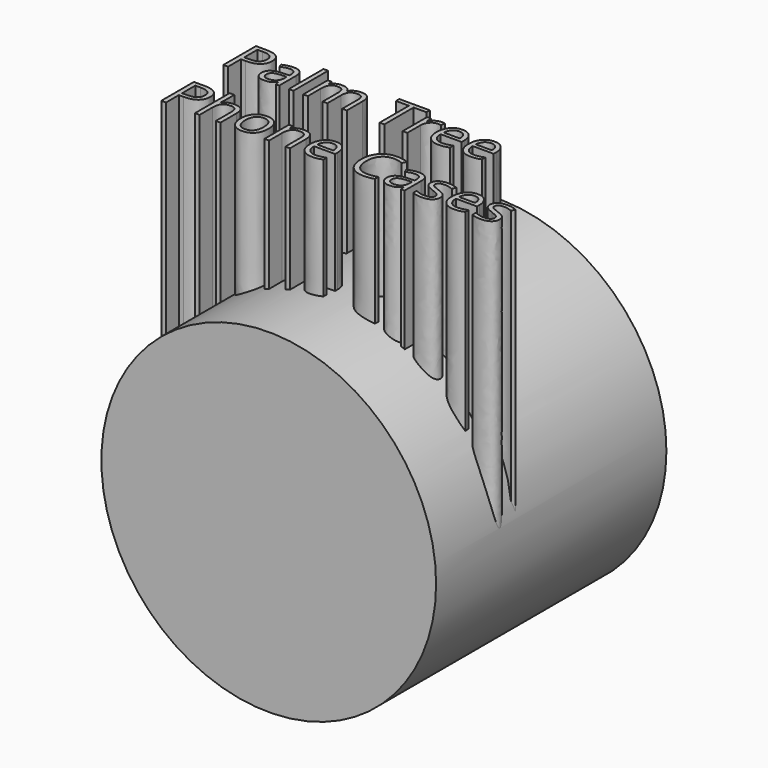
from build123d import *

# Parameters (mm, degrees)
F0_R         = 29.5338666702
F1_DEPTH     = 50.8
F2_TEXT_SIZE = 10.0707014402
F3_DEPTH     = 50.8
F4_R         = 25.9330479269
F5_DEPTH     = 50.292


# Not quite as in the source:
# - Text() gives the source's letters only with a copy of the font that has no kerning and outlines rounded to 1/6400 em; it was checked with that copy


with BuildPart() as f1:
    # F0 (on Front) → F1 (new body)
    with BuildSketch(Plane.XZ):
        Circle(F0_R)
    extrude(amount=F1_DEPTH)

    # F2 (on Top) → F3 (join)
    with BuildSketch(Plane.XY):
        with Locations((-30.1287677139, -24.378048256)):
            Text('Palm Tree', F2_TEXT_SIZE, font='Open Sans', text_align=(TextAlign.LEFT, TextAlign.BOTTOM))
        with Locations((-30.1287677139, -38.0742022147)):
            Text('Phone Cases', F2_TEXT_SIZE, font='Open Sans', text_align=(TextAlign.LEFT, TextAlign.BOTTOM))
    extrude(amount=F3_DEPTH)

    # F4 (on face) → F5 (cut)
    with BuildSketch(Plane(origin=(0, 0, 0), x_dir=(-1, 0, 0), z_dir=(0, 1, 0))):
        Circle(F4_R)
    extrude(amount=-F5_DEPTH, mode=Mode.SUBTRACT)


solid = f1.part
